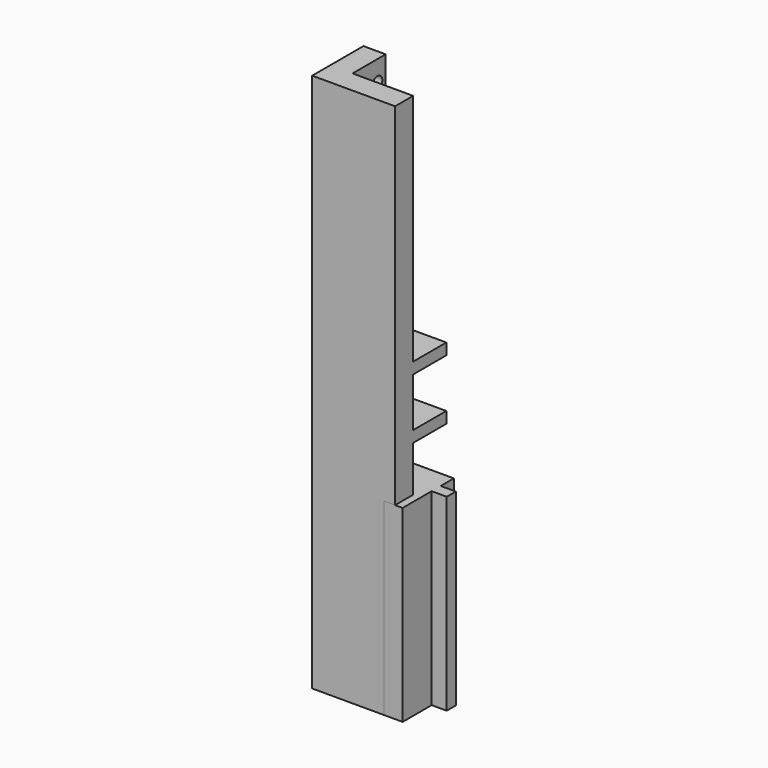
from build123d import *

# Parameters (mm, degrees)
F0_W              = 22
F0_H              = 17
F0_R              = 3
F1_DEPTH          = 71.6
F3_DEPTH          = 6.5
F4_W              = 16.1
F4_H              = 62.1
F5_DEPTH          = 11
F6_W              = 3
F6_H              = 50
F7_DEPTH          = 25
F9_D              = 3.3
F9_DEPTH          = 7
F9_TIP            = 0.9914200214
F10_R             = 3
F10_W             = 5
F10_H             = 6
F10_W_2           = 4
F10_H_2           = 3
F11_DEPTH         = 50
F13_D             = 2
F13_DEPTH         = 16
F13_CBORE_D       = 4.1
F13_CBORE_DEPTH   = 3
F13_TIP           = 0.600860619
F13_2_D           = 2
F13_2_DEPTH       = 16
F13_2_CBORE_D     = 4.1
F13_2_CBORE_DEPTH = 3
F13_2_TIP         = 0.600860619


with BuildPart() as f1:
    # F0 (on Top) → F1 (new body, symmetric)
    with BuildSketch(Plane.XY):
        with Locations((11, 8.5)):
            Rectangle(F0_W, F0_H)
        with Locations((11, 11)):
            Circle(F0_R, mode=Mode.SUBTRACT)
    extrude(amount=F1_DEPTH, both=True)

    # F2 (on Top) → F3 (cut, symmetric)
    with BuildSketch(Plane.XY):
        with BuildLine():
            ThreePointArc((11, 5.9), (14.6062445841, 7.3937554159), (16.1, 11))
            ThreePointArc((16.1, 11), (11, 16.1), (5.9, 11))
            ThreePointArc((5.9, 11), (7.3937554159, 7.3937554159), (11, 5.9))
        make_face()
        with BuildLine():
            ThreePointArc((5.9, 11), (11, 16.1), (16.1, 11))
            ThreePointArc((16.1, 11), (14.6062445841, 7.3937554159), (11, 5.9))
            Line((11, 5.9), (22, 5.9))
            Line((22, 5.9), (22, 17))
            Line((22, 17), (5.9, 17))
            Line((5.9, 17), (5.9, 11))
        make_face()
    extrude(amount=F3_DEPTH, both=True, mode=Mode.SUBTRACT)

    # F4 (on face) → F5 (cut)
    with BuildSketch(Plane(origin=(0, 17, 0), x_dir=(-1, 0, 0), z_dir=(0, 1, 0))):
        with Locations((-13.95, -40.55)):
            Rectangle(F4_W, F4_H)
        with Locations((-13.95, 40.55)):
            Rectangle(F4_W, F4_H)
    extrude(amount=-F5_DEPTH, mode=Mode.SUBTRACT)

    # F6 (on face) → F7 (cut)
    with BuildSketch(Plane(origin=(0, 6, 0), x_dir=(-1, 0, 0), z_dir=(0, 1, 0))):
        with Locations((-20.5, -46.6)):
            Rectangle(F6_W, F6_H)
    extrude(amount=-F7_DEPTH, mode=Mode.SUBTRACT)

    # F9
    with Locations(Plane(origin=(0, 0, 0), x_dir=(0, -1, 0), z_dir=(-1, 0, 0))):
        with Locations((-2.75, -66), (-14.25, 66)):
            Hole(F9_D / 2, depth=F9_DEPTH)
            with Locations((0, 0, -(F9_DEPTH + F9_TIP / 2))):  # 118° drill point
                Cone(0, F9_D / 2, F9_TIP, mode=Mode.SUBTRACT)

    # F13
    with Locations(Plane(origin=(0, 17, 0), x_dir=(-1, 0, 0), z_dir=(0, 1, 0))):
        with Locations((-15.9, -64.6), (-15.9, -52.6), (-15.9, -40.6), (-15.9, -28.6)):
            CounterBoreHole(F13_D / 2, F13_CBORE_D / 2, F13_CBORE_DEPTH, depth=F13_DEPTH)
            with Locations((0, 0, -(F13_DEPTH + F13_TIP / 2))):  # 118° drill point
                Cone(0, F13_D / 2, F13_TIP, mode=Mode.SUBTRACT)


with BuildPart() as f11:
    # F10 (on face) → F11 (new body)
    with BuildSketch(Plane(origin=(0, 0, -71.6), x_dir=(1, 0, 0), z_dir=(0, 0, -1))):
        Polygon((19, -6), (5.9, -6), (5.9, -17), (24, -17), (24, -12.6333478838), (24, -9.6333478838), (24, -6), align=None)
        with Locations((11, -11)):
            Circle(F10_R, mode=Mode.SUBTRACT)
        with Locations((21.5, -3)):
            Rectangle(F10_W, F10_H)
        with Locations((26, -11.1333478838)):
            Rectangle(F10_W_2, F10_H_2)
    extrude(amount=-F11_DEPTH)

    # F13#2
    with Locations(Plane(origin=(0, 17, 0), x_dir=(-1, 0, 0), z_dir=(0, 1, 0))):
        with Locations((-15.9, -64.6), (-15.9, -52.6), (-15.9, -40.6), (-15.9, -28.6)):
            CounterBoreHole(F13_2_D / 2, F13_2_CBORE_D / 2, F13_2_CBORE_DEPTH, depth=F13_2_DEPTH)
            with Locations((0, 0, -(F13_2_DEPTH + F13_2_TIP / 2))):  # 118° drill point
                Cone(0, F13_2_D / 2, F13_2_TIP, mode=Mode.SUBTRACT)


solid = Compound([f1.part, f11.part])
